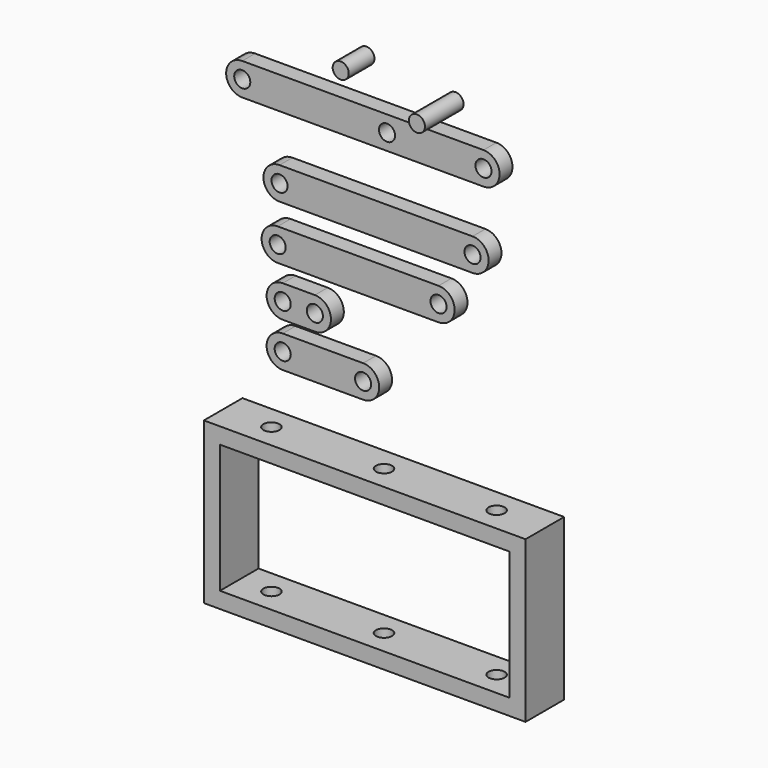
from build123d import *

# Parameters (mm, degrees)
F1_R      = 2.5
F2_DEPTH  = 5
F3_R      = 2.5
F4_DEPTH  = 5
F5_R      = 2.5
F6_DEPTH  = 5
F7_R      = 2.5
F8_DEPTH  = 5
F9_R      = 2.5
F10_DEPTH = 5
F11_W     = 100
F11_H     = 50
F11_W_2   = 90
F11_H_2   = 40
F12_DEPTH = 15
F13_R     = 2.5
F14_DEPTH = 50
F15_R     = 2.5
F16_DEPTH = 10
F17_R     = 2.5
F18_DEPTH = 15


with BuildPart() as f2:
    # F1 (on Front) → F2 (new body)
    with BuildSketch(Plane.XZ):
        with BuildLine():
            Line((10, 5), (0, 5))
            ThreePointArc((0, 5), (-5, 0), (0, -5))
            Line((0, -5), (10, -5))
            ThreePointArc((10, -5), (15, 0), (10, 5))
        make_face()
        Circle(F1_R, mode=Mode.SUBTRACT)
        with Locations((10, 0)):
            Circle(F1_R, mode=Mode.SUBTRACT)
    extrude(amount=F2_DEPTH)


with BuildPart() as f4:
    # F3 (on Front) → F4 (new body)
    with BuildSketch(Plane.XZ):
        with BuildLine():
            Line((25, -8.7587906366), (0, -8.7587906366))
            ThreePointArc((0, -8.7587906366), (-5, -13.7587906366), (0, -18.7587906366))
            Line((0, -18.7587906366), (25, -18.7587906366))
            ThreePointArc((25, -18.7587906366), (30, -13.7587906366), (25, -8.7587906366))
        make_face()
        with Locations((0, -13.7587906366)):
            Circle(F3_R, mode=Mode.SUBTRACT)
        with Locations((25, -13.7587906366)):
            Circle(F3_R, mode=Mode.SUBTRACT)
    extrude(amount=F4_DEPTH)


with BuildPart() as f6:
    # F5 (on Front) → F6 (new body)
    with BuildSketch(Plane.XZ):
        with BuildLine():
            Line((48.4452299587, 20.0459017605), (-1.5547700413, 20.0459017605))
            ThreePointArc((-1.5547700413, 20.0459017605), (-6.5547700413, 15.0459017605), (-1.5547700413, 10.0459017605))
            Line((-1.5547700413, 10.0459017605), (48.4452299587, 10.0459017605))
            ThreePointArc((48.4452299587, 10.0459017605), (53.4452299587, 15.0459017605), (48.4452299587, 20.0459017605))
        make_face()
        with Locations((-1.5547700413, 15.0459017605)):
            Circle(F5_R, mode=Mode.SUBTRACT)
        with Locations((48.4452299587, 15.0459017605)):
            Circle(F5_R, mode=Mode.SUBTRACT)
    extrude(amount=F6_DEPTH)


with BuildPart() as f8:
    # F7 (on Front) → F8 (new body)
    with BuildSketch(Plane.XZ):
        with BuildLine():
            Line((59.0105567314, 37.0056974888), (-0.9894432686, 37.0056974888))
            ThreePointArc((-0.9894432686, 37.0056974888), (-5.9894432686, 32.0056974888), (-0.9894432686, 27.0056974888))
            Line((-0.9894432686, 27.0056974888), (59.0105567314, 27.0056974888))
            ThreePointArc((59.0105567314, 27.0056974888), (64.0105567314, 32.0056974888), (59.0105567314, 37.0056974888))
        make_face()
        with Locations((-0.9894432686, 32.0056974888)):
            Circle(F7_R, mode=Mode.SUBTRACT)
        with Locations((59.0105567314, 32.0056974888)):
            Circle(F7_R, mode=Mode.SUBTRACT)
    extrude(amount=F8_DEPTH)


with BuildPart() as f10:
    # F9 (on Front) → F10 (new body)
    with BuildSketch(Plane.XZ):
        with BuildLine():
            Line((62.4213630147, 61.7387342453), (-12.5786369853, 61.7387342453))
            ThreePointArc((-12.5786369853, 61.7387342453), (-17.5786369853, 56.7387342453), (-12.5786369853, 51.7387342453))
            Line((-12.5786369853, 51.7387342453), (62.4213630147, 51.7387342453))
            ThreePointArc((62.4213630147, 51.7387342453), (67.4213630147, 56.7387342453), (62.4213630147, 61.7387342453))
        make_face()
        with Locations((-12.5786369853, 56.7387342453)):
            Circle(F9_R, mode=Mode.SUBTRACT)
        with Locations((32.4213630147, 56.7387342453)):
            Circle(F9_R, mode=Mode.SUBTRACT)
        with Locations((62.4213630147, 56.7387342453)):
            Circle(F9_R, mode=Mode.SUBTRACT)
    extrude(amount=F10_DEPTH)


with BuildPart() as f12:
    # F11 (on Front) → F12 (new body)
    with BuildSketch(Plane.XZ):
        with Locations((33.4885520861, -58.8550369338)):
            Rectangle(F11_W, F11_H)
        with Locations((33.4885520861, -58.8550369338)):
            Rectangle(F11_W_2, F11_H_2, mode=Mode.SUBTRACT)
    extrude(amount=F12_DEPTH)

    # F13 (on face) → F14 (cut)
    with BuildSketch(Plane(origin=(0, 0, -83.8550369338), x_dir=(1, 0, 0), z_dir=(0, 0, -1))):
        with Locations((-1.5114479139, 7.5)):
            Circle(F13_R)
        with Locations((33.4885520861, 7.5)):
            Circle(F13_R)
        with Locations((68.4885520861, 7.5)):
            Circle(F13_R)
    extrude(amount=-F14_DEPTH, mode=Mode.SUBTRACT)


with BuildPart() as f16:
    # F15 (on Front) → F16 (new body)
    with BuildSketch(Plane.XZ):
        with Locations((22.0284182578, 72.3978579044)):
            Circle(F15_R)
    extrude(amount=F16_DEPTH)


with BuildPart() as f18:
    # F17 (on Front) → F18 (new body)
    with BuildSketch(Plane.XZ):
        with Locations((49.7182831168, 68.9315199852)):
            Circle(F17_R)
    extrude(amount=F18_DEPTH)


solid = Compound([f2.part, f4.part, f6.part, f8.part, f10.part, f12.part, f16.part, f18.part])
